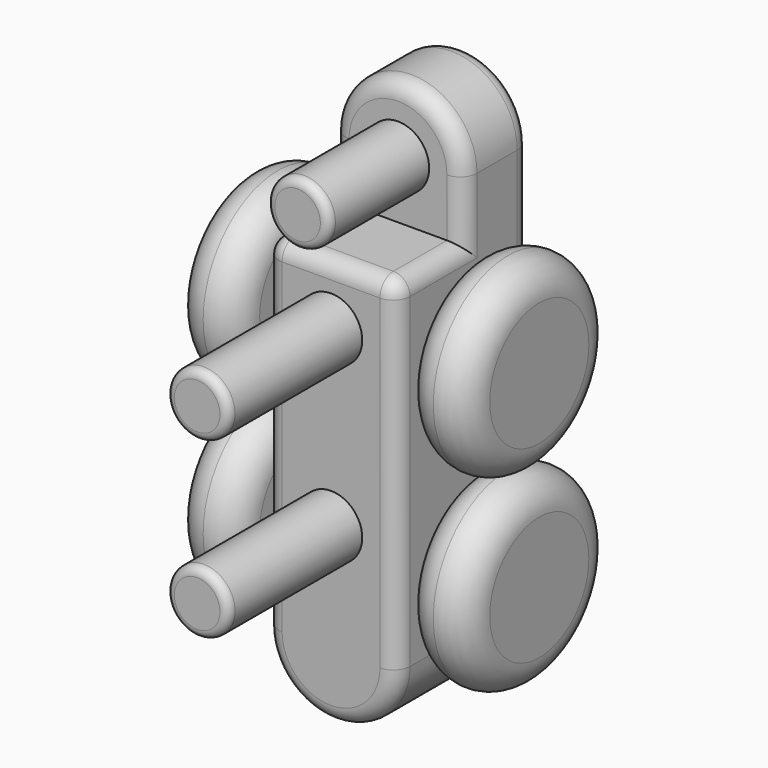
from build123d import *

# Parameters (mm, degrees)
F0_R      = 9.4597461698
F1_DEPTH  = 101.6
F0_W      = 39.8592872384
F0_H      = 103.9333879682
F2_DEPTH  = 50.8
F3_DEPTH  = 25.4
F4_DEPTH  = 63.5
F5_R      = 5.08
F6_R      = 5.08
F7_R      = 5.08
F8_R      = 8.4595796919
F9_DEPTH  = 25.4
F10_R     = 4.7404099138
F11_DEPTH = 25.4
F12_R     = 2.54
F14_R     = 28.321
F14_R_2   = 4.7404099138
F15_DEPTH = 19.05
F16_R     = 9.52499
F16_2_R   = 9.52499
F17_R     = 28.321
F17_R_2   = 4.7404099138
F18_DEPTH = 19.05
F19_R     = 9.52499
F19_2_R   = 9.52499


# Not quite as in the source:
# - a fillet or chamfer is up to 0.001 mm smaller than in the source, because OpenCascade refuses the exact size


with BuildPart() as f1:
    # F0 (on Front) → F1 (new body)
    with BuildSketch(Plane.XZ):
        with Locations((0, -35.6362370717)):
            Circle(F0_R)
    extrude(amount=F1_DEPTH)



with BuildPart() as f1b:
    # F0 (on Front) → F1, piece 2 (new body)
    with BuildSketch(Plane.XZ):
        with Locations((0, -88.4090361273)):
            Circle(F0_R)
    extrude(amount=F1_DEPTH)


with BuildPart() as f1_1:
    add(f1.part)

    add(f1b.part)  # F2 merges F1b
    # F0 (on Front) → F2 (join)
    with BuildSketch(Plane.XZ):
        with Locations((0, -69.4868988952)):
            Rectangle(F0_W, F0_H)
        with Locations((0, -88.4090361273)):
            Circle(F0_R, mode=Mode.SUBTRACT)
        with Locations((0, -35.6362370717)):
            Circle(F0_R, mode=Mode.SUBTRACT)
        with BuildLine():
            ThreePointArc((-19.9296436192, -121.4535928793), (0, -141.3832364985), (19.9296436192, -121.4535928793))
            Line((19.9296436192, -121.4535928793), (-19.9296436192, -121.4535928793))
        make_face()
    extrude(amount=F2_DEPTH)

    # F0 (on Front) → F3 (join)
    with BuildSketch(Plane.XZ):
        with BuildLine():
            Line((19.9296436192, -17.5202049111), (19.9296436192, 0))
            ThreePointArc((19.9296436192, 0), (0, 19.9296436192), (-19.9296436192, 0))
            Line((-19.9296436192, 0), (-19.9296436192, -17.5202049111))
            Line((-19.9296436192, -17.5202049111), (19.9296436192, -17.5202049111))
        make_face()
        Circle(F0_R, mode=Mode.SUBTRACT)
    extrude(amount=F3_DEPTH)

    # F0 (on Front) → F4 (join)
    with BuildSketch(Plane.XZ):
        Circle(F0_R)
    extrude(amount=F4_DEPTH)

    # F5
    f5_edges = [f1_1.edges().sort_by_distance(p)[0] for p in [
        (-19.929644, -38.1, -17.520205),
        (19.929644, -50.8, -69.486899),
        (0, -50.8, -17.520205),
        (19.929644, -38.1, -17.520205),
    ]]
    fillet(f5_edges, radius=F5_R)

    # F6
    f6_edges = [f1_1.edges().sort_by_distance(p)[0] for p in [
        (19.929644, 0, -60.726796),
        (0, 0, 19.929644),
        (-19.929644, 0, -60.726796),
        (0, 0, -141.383236),
    ]]
    fillet(f6_edges, radius=F6_R)

    # F7
    f7_edges = [f1_1.edges().sort_by_distance(p)[0] for p in [
        (-19.929644, -25.4, -8.760102),
        (-19.929644, -25.4, -20.060205),
        (0, -25.4, 19.929644),
        (19.929644, -15.24, 0),
    ]]
    fillet(f7_edges, radius=F7_R)

    # F8 (on Right) → F9 (cut, symmetric)
    with BuildSketch(Plane.YZ):
        with Locations((-27.3456163704, -42.5785966218)):
            Circle(F8_R)
        with Locations((-27.3456163704, -99.8373031616)):
            Circle(F8_R)
    extrude(amount=F9_DEPTH, both=True, mode=Mode.SUBTRACT)

    # F12
    f12_edges = [f1_1.edges().sort_by_distance(p)[0] for p in [
        (-9.459746, -101.6, -88.409036),
        (-9.459746, -101.6, -35.636237),
        (-9.459746, -63.5, 0),
    ]]
    fillet(f12_edges, radius=F12_R)


with BuildPart() as f11:
    # F10 (on Right) → F11 (new body, symmetric)
    with BuildSketch(Plane.YZ):
        with Locations((-27.3456163704, -42.5785966218)):
            Circle(F10_R)
    extrude(amount=F11_DEPTH, both=True)


with BuildPart() as f11b:
    # F10 (on Right) → F11, piece 2 (new body, symmetric)
    with BuildSketch(Plane.YZ):
        with Locations((-27.3456163704, -99.8373031616)):
            Circle(F10_R)
    extrude(amount=F11_DEPTH, both=True)


with BuildPart() as f15:
    # F14 (on face) → F15 (new body)
    with BuildSketch(Plane.YZ.offset(25.4)):
        with Locations((-27.3456163704, -42.5785966218)):
            Circle(F14_R)
        with Locations((-27.3456163704, -42.5785966218)):
            Circle(F14_R_2, mode=Mode.SUBTRACT)
        with Locations((-27.3456163704, -42.5785966218)):
            Circle(F14_R_2)
    extrude(amount=F15_DEPTH)

    # F16 (radius 9.525 in the source; OpenCascade refuses exactly that, so slightly less here)
    f16_edges = [f15.edges().sort_by_distance(p)[0] for p in [
        (44.45, -55.666616, -42.578597),
        (25.4, -55.666616, -42.578597),
    ]]
    fillet(f16_edges, radius=F16_R)


with BuildPart() as f15b:
    # F14 (on face) → F15, piece 2 (new body)
    with BuildSketch(Plane.YZ.offset(25.4)):
        with Locations((-27.3456163704, -99.8373031616)):
            Circle(F14_R)
        with Locations((-27.3456163704, -99.8373031616)):
            Circle(F14_R_2, mode=Mode.SUBTRACT)
        with Locations((-27.3456163704, -99.8373031616)):
            Circle(F14_R_2)
    extrude(amount=F15_DEPTH)

    # F16#2 (radius 9.525 in the source; OpenCascade refuses exactly that, so slightly less here)
    f16_2_edges = [f15b.edges().sort_by_distance(p)[0] for p in [
        (44.45, -55.666616, -99.837303),
        (25.4, -55.666616, -99.837303),
    ]]
    fillet(f16_2_edges, radius=F16_2_R)


with BuildPart() as f18:
    # F17 (on face) → F18 (new body)
    with BuildSketch(Plane(origin=(-25.4, 0, 0), x_dir=(0, -1, 0), z_dir=(-1, 0, 0))):
        with Locations((27.3456163704, -42.5785966218)):
            Circle(F17_R)
        with Locations((27.3456163704, -42.5785966218)):
            Circle(F17_R_2, mode=Mode.SUBTRACT)
        with Locations((27.3456163704, -42.5785966218)):
            Circle(F17_R_2)
    extrude(amount=F18_DEPTH)

    # F19 (radius 9.525 in the source; OpenCascade refuses exactly that, so slightly less here)
    f19_edges = [f18.edges().sort_by_distance(p)[0] for p in [
        (-44.45, 0.975384, -42.578597),
        (-25.4, 0.975384, -42.578597),
    ]]
    fillet(f19_edges, radius=F19_R)


with BuildPart() as f18b:
    # F17 (on face) → F18, piece 2 (new body)
    with BuildSketch(Plane(origin=(-25.4, 0, 0), x_dir=(0, -1, 0), z_dir=(-1, 0, 0))):
        with Locations((27.3456163704, -99.8373031616)):
            Circle(F17_R)
        with Locations((27.3456163704, -99.8373031616)):
            Circle(F17_R_2, mode=Mode.SUBTRACT)
        with Locations((27.3456163704, -99.8373031616)):
            Circle(F17_R_2)
    extrude(amount=F18_DEPTH)

    # F19#2 (radius 9.525 in the source; OpenCascade refuses exactly that, so slightly less here)
    f19_2_edges = [f18b.edges().sort_by_distance(p)[0] for p in [
        (-44.45, 0.975384, -99.837303),
        (-25.4, 0.975384, -99.837303),
    ]]
    fillet(f19_2_edges, radius=F19_2_R)


solid = Compound([f1_1.part, f11.part, f11b.part, f15.part, f15b.part, f18.part, f18b.part])
